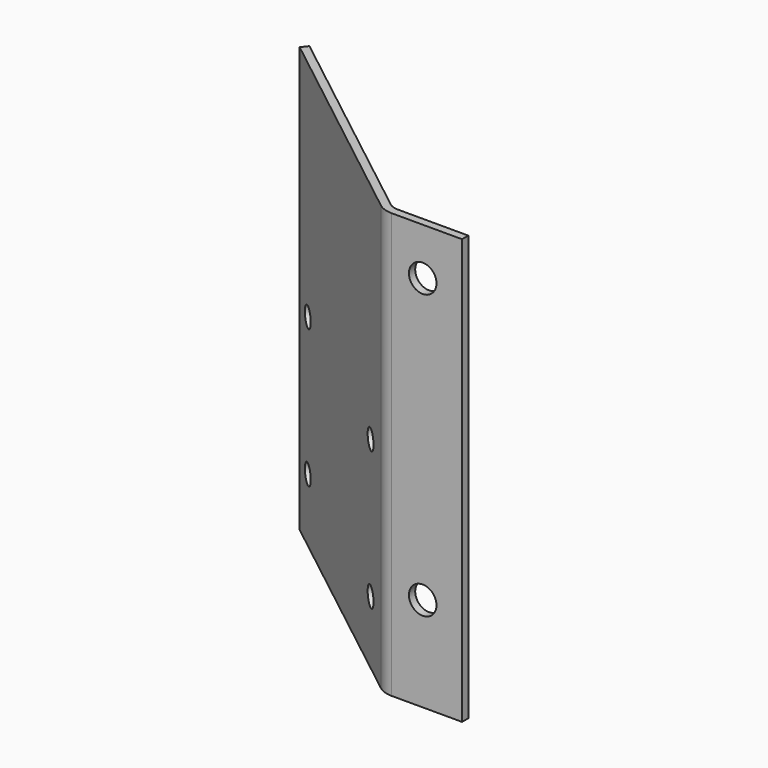
from build123d import *

# Parameters (mm, degrees)
F1_DEPTH = 171.45
F2_R     = 5.5626
F3_DEPTH = 72.8730407724
F4_R     = 3.9751
F5_DEPTH = 76.9722036075


# Not quite as in the source:
# - a feature of the source that left no trace in its solid (it failed there, or was rolled back) is left out


with BuildPart() as f1:
    # F0 (on Top) → F1 (new body)
    with BuildSketch(Plane.XY):
        with BuildLine():
            Line((0, -3.175), (0, 0))
            Line((0, 0), (-28.4702794834, 0))
            ThreePointArc((-28.4702794834, 0), (-30.5376372642, 0.3459570449), (-32.3797298517, 1.3461317146))
            Line((-32.3797298517, 1.3461317146), (-119.8649039531, 69.6970407724))
            Line((-119.8649039531, 69.6970407724), (-121.8196291372, 67.1951066297))
            Line((-121.8196291372, 67.1951066297), (-34.3344550359, -1.1558024281))
            ThreePointArc((-34.3344550359, -1.1558024281), (-31.5713161546, -2.6560644326), (-28.4702794834, -3.175))
            Line((-28.4702794834, -3.175), (0, -3.175))
        make_face()
    extrude(amount=F1_DEPTH)

    # F2 (on face) → F3 (cut, through all)
    with BuildSketch(Plane.XZ.offset(3.175)):
        with Locations((-15.875, 152.4)):
            Circle(F2_R)
        with Locations((-15.875, 38.1)):
            Circle(F2_R)
    extrude(amount=-F3_DEPTH, mode=Mode.SUBTRACT)

    # F4 (on face) → F5 (cut, through all)
    with BuildSketch(Plane(origin=(-13.5748343728, -17.3749956639, 0), x_dir=(0.7880107536, -0.6156614753, 0), z_dir=(-0.6156614753, -0.7880107536, 0))):
        with Locations((-126.2394162429, 81.28)):
            Circle(F4_R)
        with Locations((-40.5144162429, 81.28)):
            Circle(F4_R)
        with Locations((-40.5144162429, 25.4)):
            Circle(F4_R)
        with Locations((-126.2394162429, 25.4)):
            Circle(F4_R)
    extrude(amount=-F5_DEPTH, mode=Mode.SUBTRACT)


solid = f1.part
